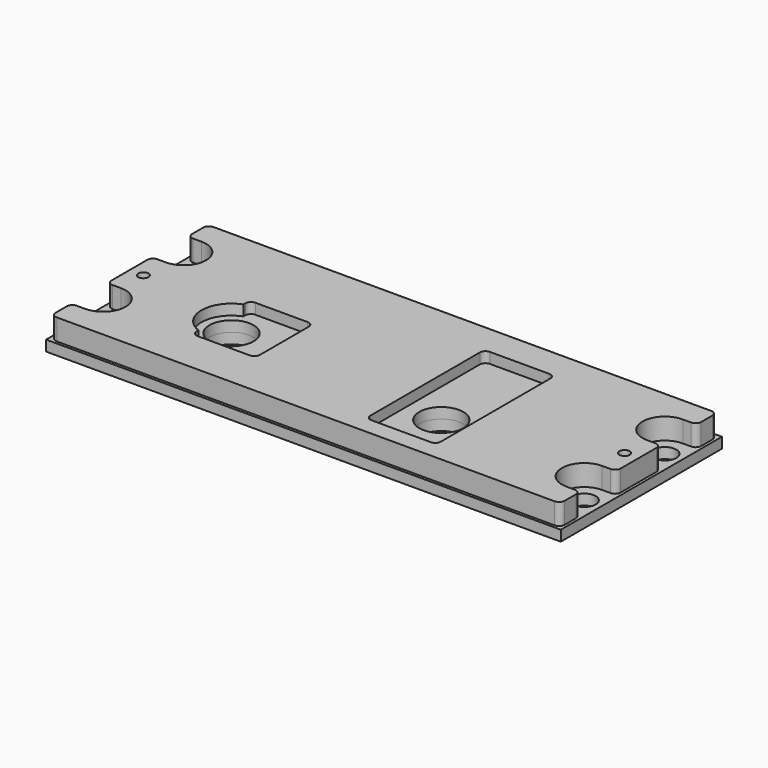
from build123d import *

# Parameters (mm, degrees)
F0_W        = 146.05
F0_H        = 57.15
F0_R        = 3.24
F1_DEPTH    = 3
F2_DEPTH    = 6
F3_R        = 1.588
F5_W        = 20
F5_H        = 42
F5_R        = 6.25
F6_DEPTH    = 3
F7_DEPTH    = 25
F8_R        = 1.588
F10_D       = 2.9
F10_DEPTH   = 10
F10_TIP     = 0.8712478976
F10_2_D     = 2.9
F10_2_DEPTH = 10
F10_2_TIP   = 0.8712478976


with BuildPart() as f1:
    # F0 (on Top) → F1 (new body)
    with BuildSketch(Plane.XY):
        Rectangle(F0_W, F0_H)
        with Locations((-68.2625, -14.287)):
            Circle(F0_R, mode=Mode.SUBTRACT)
        with Locations((68.2625, -14.287)):
            Circle(F0_R, mode=Mode.SUBTRACT)
        with Locations((-68.2625, 14.287)):
            Circle(F0_R, mode=Mode.SUBTRACT)
        with BuildLine():
            Line((-72.225, 27.775), (72.225, 27.775))
            Line((72.225, 27.775), (72.225, 20.6375))
            Line((72.225, 20.6375), (68.2625, 20.6375))
            ThreePointArc((68.2625, 20.6375), (61.912, 14.287), (68.2625, 7.9365))
            Line((68.2625, 7.9365), (72.225, 7.9365))
            Line((72.225, 7.9365), (72.225, -7.9365))
            Line((72.225, -7.9365), (68.2625, -7.9365))
            ThreePointArc((68.2625, -7.9365), (61.912, -14.287), (68.2625, -20.6375))
            Line((68.2625, -20.6375), (72.225, -20.6375))
            Line((72.225, -20.6375), (72.225, -27.775))
            Line((72.225, -27.775), (-72.225, -27.775))
            Line((-72.225, -27.775), (-72.225, -20.6375))
            Line((-72.225, -20.6375), (-68.2625, -20.6375))
            ThreePointArc((-68.2625, -20.6375), (-61.912, -14.287), (-68.2625, -7.9365))
            Line((-68.2625, -7.9365), (-72.225, -7.9365))
            Line((-72.225, -7.9365), (-72.225, 7.9365))
            Line((-72.225, 7.9365), (-68.2625, 7.9365))
            ThreePointArc((-68.2625, 7.9365), (-61.912, 14.287), (-68.2625, 20.6375))
            Line((-68.2625, 20.6375), (-72.225, 20.6375))
            Line((-72.225, 20.6375), (-72.225, 27.775))
        make_face(mode=Mode.SUBTRACT)
        with Locations((68.2625, 14.287)):
            Circle(F0_R, mode=Mode.SUBTRACT)
        with BuildLine():
            Line((72.225, 20.6375), (72.225, 27.775))
            Line((72.225, 27.775), (-72.225, 27.775))
            Line((-72.225, 27.775), (-72.225, 20.6375))
            Line((-72.225, 20.6375), (-68.2625, 20.6375))
            ThreePointArc((-68.2625, 20.6375), (-61.912, 14.287), (-68.2625, 7.9365))
            Line((-68.2625, 7.9365), (-72.225, 7.9365))
            Line((-72.225, 7.9365), (-72.225, -7.9365))
            Line((-72.225, -7.9365), (-68.2625, -7.9365))
            ThreePointArc((-68.2625, -7.9365), (-61.912, -14.287), (-68.2625, -20.6375))
            Line((-68.2625, -20.6375), (-72.225, -20.6375))
            Line((-72.225, -20.6375), (-72.225, -27.775))
            Line((-72.225, -27.775), (72.225, -27.775))
            Line((72.225, -27.775), (72.225, -20.6375))
            Line((72.225, -20.6375), (68.2625, -20.6375))
            ThreePointArc((68.2625, -20.6375), (61.912, -14.287), (68.2625, -7.9365))
            Line((68.2625, -7.9365), (72.225, -7.9365))
            Line((72.225, -7.9365), (72.225, 7.9365))
            Line((72.225, 7.9365), (68.2625, 7.9365))
            ThreePointArc((68.2625, 7.9365), (61.912, 14.287), (68.2625, 20.6375))
            Line((68.2625, 20.6375), (72.225, 20.6375))
        make_face()
    extrude(amount=-F1_DEPTH)


with BuildPart() as f2:
    # F0 (on Top) → F2 (new body)
    with BuildSketch(Plane.XY):
        with BuildLine():
            Line((72.225, 20.6375), (72.225, 27.775))
            Line((72.225, 27.775), (-72.225, 27.775))
            Line((-72.225, 27.775), (-72.225, 20.6375))
            Line((-72.225, 20.6375), (-68.2625, 20.6375))
            ThreePointArc((-68.2625, 20.6375), (-61.912, 14.287), (-68.2625, 7.9365))
            Line((-68.2625, 7.9365), (-72.225, 7.9365))
            Line((-72.225, 7.9365), (-72.225, -7.9365))
            Line((-72.225, -7.9365), (-68.2625, -7.9365))
            ThreePointArc((-68.2625, -7.9365), (-61.912, -14.287), (-68.2625, -20.6375))
            Line((-68.2625, -20.6375), (-72.225, -20.6375))
            Line((-72.225, -20.6375), (-72.225, -27.775))
            Line((-72.225, -27.775), (72.225, -27.775))
            Line((72.225, -27.775), (72.225, -20.6375))
            Line((72.225, -20.6375), (68.2625, -20.6375))
            ThreePointArc((68.2625, -20.6375), (61.912, -14.287), (68.2625, -7.9365))
            Line((68.2625, -7.9365), (72.225, -7.9365))
            Line((72.225, -7.9365), (72.225, 7.9365))
            Line((72.225, 7.9365), (68.2625, 7.9365))
            ThreePointArc((68.2625, 7.9365), (61.912, 14.287), (68.2625, 20.6375))
            Line((68.2625, 20.6375), (72.225, 20.6375))
        make_face()
    extrude(amount=F2_DEPTH)

    # F3
    f3_edges = [f2.edges().sort_by_distance(p)[0] for p in [
        (-72.225, 27.775, 3),
        (-72.225, 20.6375, 3),
        (-72.225, 7.9365, 3),
        (-72.225, -7.9365, 3),
        (-72.225, -20.6375, 3),
        (-72.225, -27.775, 3),
        (72.225, 20.6375, 3),
        (72.225, -7.9365, 3),
        (72.225, -27.775, 3),
        (72.225, -20.6375, 3),
        (72.225, 7.9365, 3),
        (72.225, 27.775, 3),
    ]]
    fillet(f3_edges, radius=F3_R)

    # F5 (on face) → F6 (cut)
    with BuildSketch(Plane.XY.offset(6)):
        with Locations((23.0761349574, -1.7581597865)):
            Rectangle(F5_W, F5_H)
        with Locations((23.0761349574, -8.5081597865)):
            Circle(F5_R, mode=Mode.SUBTRACT)
        with BuildLine():
            Line((-42.2436161637, 5.2037057467), (-42.2436161637, 2.906692607))
            ThreePointArc((-42.2436161637, 2.906692607), (-47.7436161637, -5.0462942533), (-42.2436161637, -12.9992811136))
            Line((-42.2436161637, -12.9992811136), (-42.2436161637, -15.2962942533))
            Line((-42.2436161637, -15.2962942533), (-24.2436161637, -15.2962942533))
            Line((-24.2436161637, -15.2962942533), (-24.2436161637, 5.2037057467))
            Line((-24.2436161637, 5.2037057467), (-42.2436161637, 5.2037057467))
        make_face()
        with Locations((-39.2436161637, -5.0462942533)):
            Circle(F5_R, mode=Mode.SUBTRACT)
    extrude(amount=-F6_DEPTH, mode=Mode.SUBTRACT)


with BuildPart() as f7_tool:
    # F5 (on face) → F7 (new body)
    with BuildSketch(Plane.XY.offset(6)):
        with Locations((23.0761349574, -8.5081597865)):
            Circle(F5_R)
        with Locations((-39.2436161637, -5.0462942533)):
            Circle(F5_R)
    extrude(amount=-F7_DEPTH)


with BuildPart() as f1_1:
    add(f1.part)

    # F7: cut by f7_tool
    add(f7_tool.part, mode=Mode.SUBTRACT)

    # F10
    with Locations(Plane.XY.offset(6)):
        with Locations((-68.2625, 0), (68.2625, 0)):
            Hole(F10_D / 2, depth=F10_DEPTH)
            with Locations((0, 0, -(F10_DEPTH + F10_TIP / 2))):  # 118° drill point
                Cone(0, F10_D / 2, F10_TIP, mode=Mode.SUBTRACT)


with BuildPart() as f2_1:
    add(f2.part)

    # F7: cut by f7_tool
    add(f7_tool.part, mode=Mode.SUBTRACT)

    # F8
    f8_edges = [f2_1.edges().sort_by_distance(p)[0] for p in [
        (-42.243616, 5.203706, 4.5),
        (-24.243616, 5.203706, 4.5),
        (-24.243616, -15.296294, 4.5),
        (13.076135, 19.24184, 4.5),
        (33.076135, 19.24184, 4.5),
        (13.076135, -22.75816, 4.5),
        (33.076135, -22.75816, 4.5),
        (-42.243616, -15.296294, 4.5),
    ]]
    fillet(f8_edges, radius=F8_R)

    # F10#2
    with Locations(Plane.XY.offset(6)):
        with Locations((-68.2625, 0), (68.2625, 0)):
            Hole(F10_2_D / 2, depth=F10_2_DEPTH)
            with Locations((0, 0, -(F10_2_DEPTH + F10_2_TIP / 2))):  # 118° drill point
                Cone(0, F10_2_D / 2, F10_2_TIP, mode=Mode.SUBTRACT)


solid = Compound([f1_1.part, f2_1.part])
